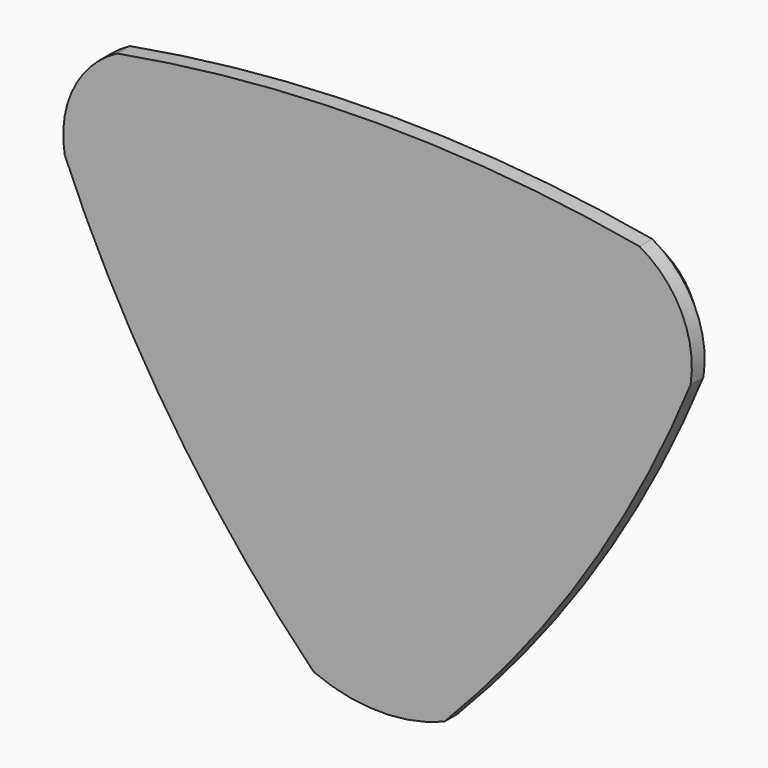
from build123d import *

# Parameters (mm, degrees)
F1_DEPTH   = 11.684
F2_C1_SIZE = 7.62
F2_C2_SIZE = 7.62
F2_C3_SIZE = 7.62
F2_C4_SIZE = 7.62
F2_C5_SIZE = 7.62
F2_C6_SIZE = 7.62


with BuildPart() as f1:
    # F0 (on Front) → F1 (new body)
    with BuildSketch(Plane.XZ):
        with BuildLine():
            ThreePointArc((79.3173238635, 29.9024358392), (77.0284346929, 45.2852812744), (66.3258507848, 56.569147855))
            ThreePointArc((66.3258507848, 56.569147855), (0.0009424984, 62.4915389193), (-66.3239657879, 56.569147855))
            ThreePointArc((-66.3239657879, 56.569147855), (-77.3864565896, 45.2349353182), (-79.657331109, 29.5605547726))
            ThreePointArc((-79.657331109, 29.5605547726), (-52.5977791189, -20.9983919929), (-16.4093449712, -65.4823631048))
            ThreePointArc((-16.4093449712, -65.4823631048), (0.1379989143, -68.9400736173), (16.753109172, -65.8242329955))
            ThreePointArc((16.753109172, -65.8242329955), (52.5805254234, -20.9315825649), (79.3173238635, 29.9024358392))
        make_face()
    extrude(amount=F1_DEPTH)

    # F2: chamfer of 7.62 on 6 edges, made by hand

    # F2_c1
    f2_c1_edges = [f1.edges().sort_by_distance(p)[0] for p in [
        (0.0009424984, 0, 62.4915389193),
    ]]
    chamfer(f2_c1_edges, length=F2_C1_SIZE)

    # F2_c2
    f2_c2_edges = [f1.edges().sort_by_distance(p)[0] for p in [
        (52.5805254234, 0, -20.9315825649),
    ]]
    chamfer(f2_c2_edges, length=F2_C2_SIZE)

    # F2_c3
    f2_c3_edges = [f1.edges().sort_by_distance(p)[0] for p in [
        (-52.5977791189, 0, -20.9983919929),
    ]]
    chamfer(f2_c3_edges, length=F2_C3_SIZE)

    # F2_c4
    f2_c4_edges = [f1.edges().sort_by_distance(p)[0] for p in [
        (0.4420771354, 0, -68.9421447146),
    ]]
    chamfer(f2_c4_edges, length=F2_C4_SIZE)

    # F2_c5
    f2_c5_edges = [f1.edges().sort_by_distance(p)[0] for p in [
        (-77.0468164212, 0, 45.8983976097),
    ]]
    chamfer(f2_c5_edges, length=F2_C5_SIZE)

    # F2_c6
    f2_c6_edges = [f1.edges().sort_by_distance(p)[0] for p in [
        (76.633600388, 0, 46.0621814234),
    ]]
    chamfer(f2_c6_edges, length=F2_C6_SIZE)


solid = f1.part
